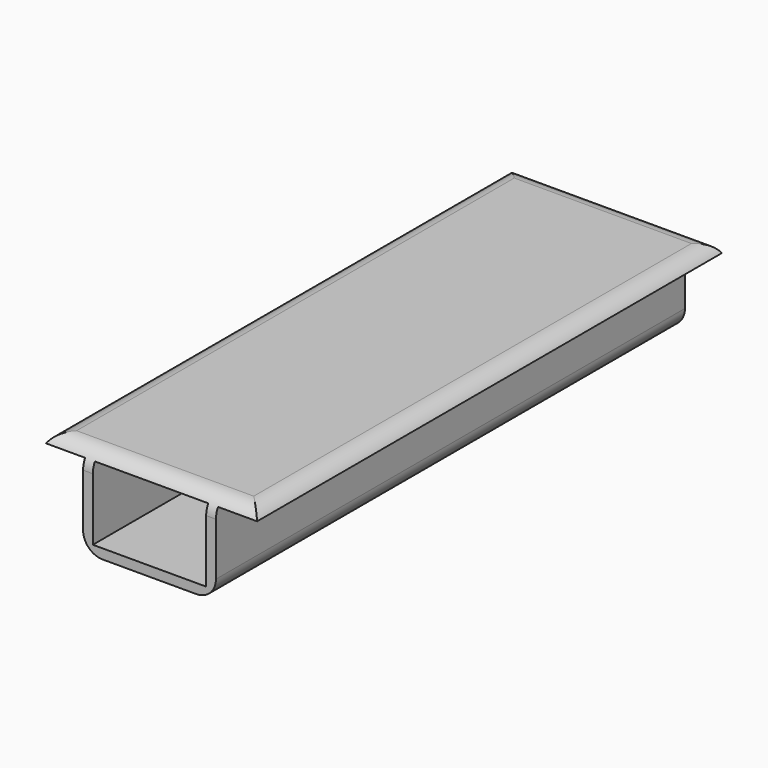
from build123d import *

# Parameters (mm, degrees)
F0_W        = 2.5
F0_H        = 18.5
F1_DEPTH    = 150
F2_T1_DEPTH = 175
F2_T3_DEPTH = 171.6506350946
F2_T5_DEPTH = 79


# Not quite as in the source:
# - a fillet or chamfer that OpenCascade refuses, or shapes differently, is made with other operations: its cross-section is extruded or revolved along the edge and cut away or added


with BuildPart() as f1:
    # F0 (on Front) → F1 (new body)
    with BuildSketch(Plane.XZ):
        Polygon((-27, 0), (-17, 0), (-14.5, 0), (-14.5, 2.5), (-27, 2.5), align=None)
        Polygon((-14.5, 2.5), (-14.5, 0), (-11, 0), (0, 0), (0, 2.5), align=None)
        with Locations((-15.75, -9.25)):
            Rectangle(F0_W, F0_H)
        Polygon((-17, -21), (0, -21), (0, -18.5), (-14.5, -18.5), (-17, -18.5), align=None)
        Polygon((0, -18.5), (0, -21), (17, -21), (17, -18.5), (14.5, -18.5), align=None)
        with Locations((15.75, -9.25)):
            Rectangle(F0_W, F0_H)
        Polygon((14.5, 2.5), (14.5, 0), (17, 0), (27, 0), (27, 2.5), align=None)
        Polygon((11, 0), (14.5, 0), (14.5, 2.5), (0, 2.5), (0, 0), align=None)
    extrude(amount=F1_DEPTH)

    # F2: fillet of radius 5 on 6 edges, made by hand

    # F2_s2 → F2_t1 (cut)
    with BuildSketch(Plane.XZ.offset(-12.5)):
        with BuildLine():
            ThreePointArc((-17, -16), (-15.5355339059, -19.5355339059), (-12, -21))
            Line((-12, -21), (-17, -21))
            Line((-17, -21), (-17, -16))
        make_face()
        with BuildLine():
            ThreePointArc((12, -21), (15.5355339059, -19.5355339059), (17, -16))
            Line((17, -16), (17, -21))
            Line((17, -21), (12, -21))
        make_face()
    extrude(amount=F2_T1_DEPTH, mode=Mode.SUBTRACT)

    # F2_s4 → F2_t3 (cut)
    with BuildSketch(Plane.XZ.offset(-10.8253175473)):
        with BuildLine():
            ThreePointArc((-22.6698729811, 2.5), (-25.1698729811, 1.8301270189), (-27, 0))
            Line((-27, 0), (-27, 2.5))
            Line((-27, 2.5), (-22.6698729811, 2.5))
        make_face()
        with BuildLine():
            ThreePointArc((27, 0), (25.1698729811, 1.8301270189), (22.6698729811, 2.5))
            Line((22.6698729811, 2.5), (27, 2.5))
            Line((27, 2.5), (27, 0))
        make_face()
    extrude(amount=F2_T3_DEPTH, mode=Mode.SUBTRACT)

    # F2_s6 → F2_t5 (cut)
    with BuildSketch(Plane.YZ.offset(-39.5)):
        with BuildLine():
            ThreePointArc((-145, 2.5), (-148.5355339059, 1.0355339059), (-150, -2.5))
            Line((-150, -2.5), (-150, 2.5))
            Line((-150, 2.5), (-145, 2.5))
        make_face()
        with BuildLine():
            ThreePointArc((-5, 2.5), (-1.4644660941, 1.0355339059), (0, -2.5))
            Line((0, -2.5), (0, 2.5))
            Line((0, 2.5), (-5, 2.5))
        make_face()
    extrude(amount=F2_T5_DEPTH, mode=Mode.SUBTRACT)


solid = f1.part
